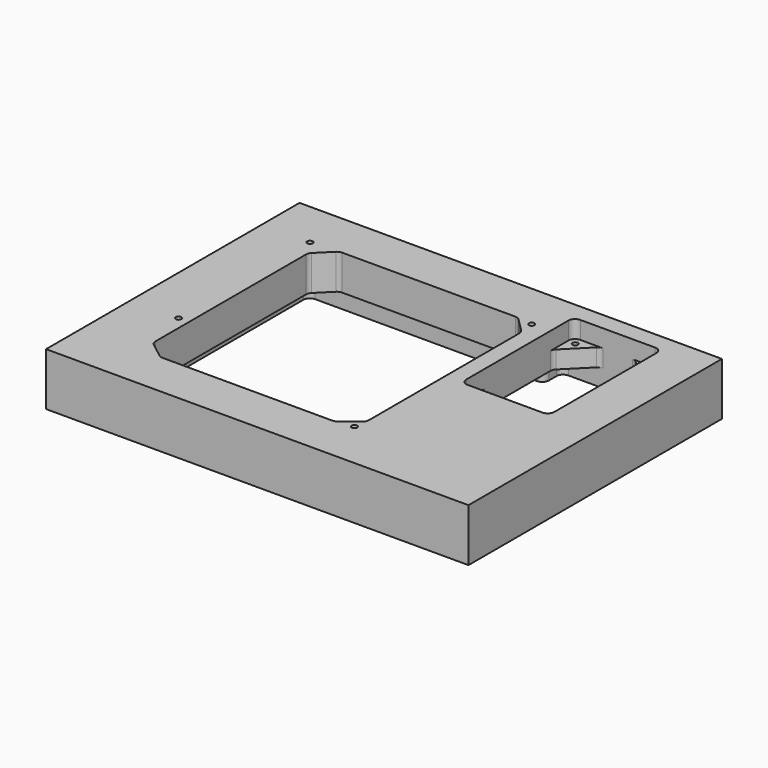
from build123d import *

# Parameters (mm, degrees)
F0_W      = 609.6
F0_H      = 457.2
F1_DEPTH  = 76.2
F3_DEPTH  = 76.201
F5_D      = 8
F6_W      = 127
F6_H      = 203.2
F7_DEPTH  = 25.4
F9_DEPTH  = 76.201
F11_DEPTH = 25.4
F12_R     = 9.525
F14_D     = 7.9375
F16_D     = 7.9375
F16_DEPTH = 12.7
F16_TIP   = 2.3846655818


# Not quite as in the source:
# - a feature names something its author has since deleted; it is built from what else it names


with BuildPart() as f1:
    # F0 (on Top) → F1 (new body)
    with BuildSketch(Plane.XY):
        with Locations((304.8, -228.6)):
            Rectangle(F0_W, F0_H)
    extrude(amount=-F1_DEPTH)

    # F2 (on Top) → F3 (cut, through all)
    with BuildSketch(Plane.XY):
        Polygon((392.35, -89.85), (367.35, -64.85), (109.35, -64.85), (84.35, -89.85), (84.35, -369.85), (112.35, -391.85), (364.35, -391.85), (392.35, -369.85), align=None)
    extrude(amount=-F3_DEPTH, mode=Mode.SUBTRACT)

    # F5 (through all)
    with Locations(Plane.XY):
        with Locations((69.35, -67.85), (389.35, -67.85), (389.35, -387.85), (69.35, -304.85)):
            Hole(F5_D / 2)

    # F6 (on Top) → F7 (cut)
    with BuildSketch(Plane.XY):
        with Locations((479.525, -127)):
            Rectangle(F6_W, F6_H)
    extrude(amount=-F7_DEPTH, mode=Mode.SUBTRACT)

    # F8 (on Top) → F9 (cut, through all)
    with BuildSketch(Plane.XY):
        Polygon((454.125, -25.4), (416.025, -63.5), (416.025, -190.5), (454.125, -228.6), (504.925, -228.6), (543.025, -190.5), (543.025, -63.5), (504.925, -25.4), align=None)
    extrude(amount=-F9_DEPTH, mode=Mode.SUBTRACT)

    # F10 (on face) → F11 (cut)
    with BuildSketch(Plane(origin=(0, 0, -76.2), x_dir=(1, 0, 0), z_dir=(0, 0, -1))):
        Polygon((398.875, 25.4), (416.025, 25.4), (543.025, 25.4), (543.025, 228.6), (416.025, 228.6), (398.875, 228.6), (398.875, 397.375), (59.825, 397.375), (59.825, 58.325), (398.875, 58.325), align=None)
    extrude(amount=-F11_DEPTH, mode=Mode.SUBTRACT)

    # F12
    f12_edges = [f1.edges().sort_by_distance(p)[0] for p in [
        (364.35, -391.85, -25.4),
        (392.35, -369.85, -25.4),
        (392.35, -89.85, -25.4),
        (367.35, -64.85, -25.4),
        (109.35, -64.85, -25.4),
        (84.35, -89.85, -25.4),
        (84.35, -369.85, -25.4),
        (112.35, -391.85, -25.4),
        (59.825, -397.375, -63.5),
        (59.825, -58.325, -63.5),
        (398.875, -58.325, -63.5),
        (398.875, -25.4, -63.5),
        (543.025, -25.4, -63.5),
        (543.025, -228.6, -63.5),
        (398.875, -228.6, -63.5),
        (398.875, -397.375, -63.5),
        (454.125, -228.6, -38.1),
        (416.025, -190.5, -38.1),
        (504.925, -228.6, -38.1),
        (543.025, -190.5, -38.1),
        (416.025, -63.5, -38.1),
        (454.125, -25.4, -38.1),
        (504.925, -25.4, -38.1),
        (543.025, -63.5, -38.1),
        (416.025, -25.4, -12.7),
        (543.025, -25.4, -12.7),
        (416.025, -228.6, -12.7),
        (543.025, -228.6, -12.7),
    ]]
    fillet(f12_edges, radius=F12_R)

    # F14 (through all)
    with Locations(Plane.XY):
        with Locations((427.1375, -36.5125), (531.9125, -36.5125), (531.9125, -217.4875), (427.1375, -217.4875)):
            Hole(F14_D / 2)

    # F16
    with Locations(Plane(origin=(0, 0, -76.2), x_dir=(1, 0, 0), z_dir=(0, 0, -1))):
        with Locations((34.925, 422.275), (574.675, 422.275), (574.675, 34.925), (34.925, 34.925)):
            Hole(F16_D / 2, depth=F16_DEPTH)
            with Locations((0, 0, -(F16_DEPTH + F16_TIP / 2))):  # 118° drill point
                Cone(0, F16_D / 2, F16_TIP, mode=Mode.SUBTRACT)


solid = f1.part
